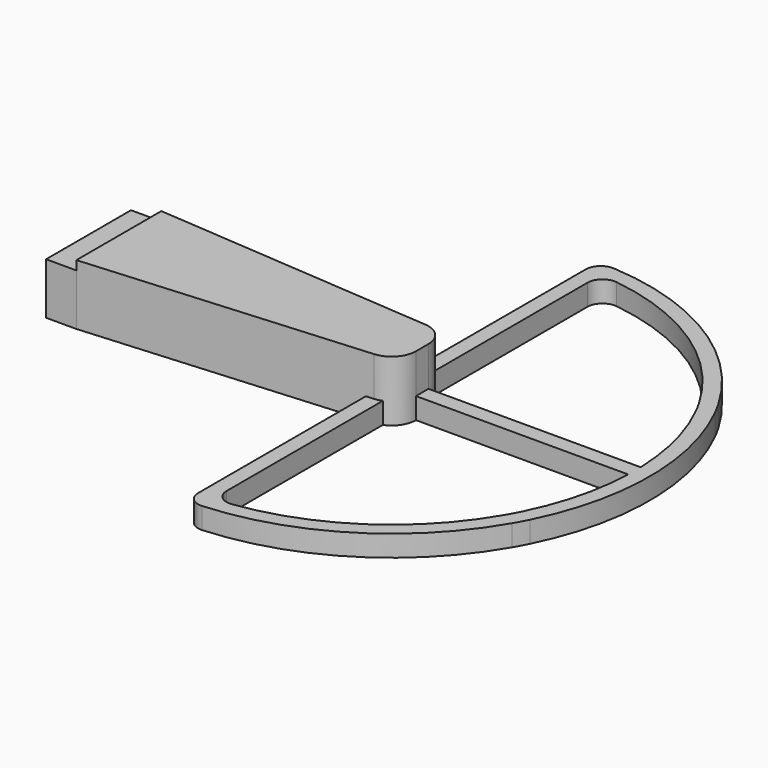
from build123d import *

# Parameters (mm, degrees)
F1_DEPTH = 10
F2_DEPTH = 17
F3_W     = 100
F3_H     = 35
F4_DEPTH = 3
F5_SIZE2 = 99.99999
F5_SIZE  = 7.49999
F6_R     = 8
F8_DEPTH = 7
F9_W     = 5.1550631039
F9_H     = 7


# Not quite as in the source:
# - a fillet or chamfer is up to 0.001 mm smaller than in the source, because OpenCascade refuses the exact size


with BuildPart() as f1:
    # F0 (on Top) → F1 (new body)
    with BuildSketch(Plane.XY):
        Polygon((-58.5, -8.5), (-58.5, -2.5), (-58.5, 0), (-58.5, 2.5), (-58.5, 8.5), (-63.5, 0), align=None)
        Polygon((-58.5, -2.5), (-55, -2.5), (-55, 2.5), (-58.5, 2.5), (-58.5, 0), align=None)
    extrude(amount=F1_DEPTH)

    # F0 (on Top) → F2 (join)
    with BuildSketch(Plane.XY):
        Polygon((-55, -17.5), (55, -17.5), (55, 17.5), (-55, 17.5), (-55, 2.5), (-55, -2.5), align=None)
    extrude(amount=F2_DEPTH)

    # F3 (on face) → F4 (join)
    with BuildSketch(Plane.XY.offset(17)):
        with Locations((5, 0)):
            Rectangle(F3_W, F3_H)
    extrude(amount=F4_DEPTH)

    # F5 (size 7.5 and 100 in the source; OpenCascade refuses exactly that, so slightly less here)
    f5_edges = [f1.edges().sort_by_distance(p)[0] for p in [
        (55, -17.5, 10),
        (55, 17.5, 10),
    ]]
    f5_side = f1.faces().sort_by_distance((55, 0, 10))[0]
    chamfer(f5_edges, length=F5_SIZE, length2=F5_SIZE2, reference=f5_side)

    # F6
    f6_edges = [f1.edges().sort_by_distance(p)[0] for p in [
        (55, -10.00001, 10),
        (55, 10.00001, 10),
    ]]
    fillet(f6_edges, radius=F6_R)

    # F7 (on face) → F8 (join)
    with BuildSketch(Plane.XY):
        with BuildLine():
            ThreePointArc((118.6121593217, 42.5), (89.7807277981, 72.2473973087), (50.3125, 84.8338219329))
            ThreePointArc((50.3125, 84.8338219329), (46.5767340156, 83.4879420476), (45, 79.8435971134))
            Line((45, 79.8435971134), (45, 0))
            Line((45, 0), (50, 2.8867513459))
            Line((50, 2.8867513459), (50, 74.3303437366))
            ThreePointArc((50, 74.3303437366), (51.708597057, 78.0942070001), (55.6666666667, 79.2856999857))
            ThreePointArc((55.6666666667, 79.2856999857), (89.5397594579, 66.4545696505), (114.2820323028, 40))
            Line((114.2820323028, 40), (118.6121593217, 42.5))
        make_face()
        with BuildLine():
            ThreePointArc((120.9846922835, 38.0962798523), (119.8308271392, 40.3155963576), (118.6121593217, 42.5))
            Line((118.6121593217, 42.5), (114.2820323028, 40))
            ThreePointArc((114.2820323028, 40), (115.4987732023, 37.8143223789), (116.6465834297, 35.5916715378))
            Line((116.6465834297, 35.5916715378), (120.9846922835, 38.0962798523))
        make_face()
        with BuildLine():
            ThreePointArc((120.9846922835, -38.0962798523), (130, 0), (120.9846922835, 38.0962798523))
            Line((120.9846922835, 38.0962798523), (116.6465834297, 35.5916715378))
            ThreePointArc((116.6465834297, 35.5916715378), (125, 0), (116.6465834297, -35.5916715378))
            Line((116.6465834297, -35.5916715378), (120.9846922835, -38.0962798523))
        make_face()
        with BuildLine():
            Line((50, -2.8867513459), (45, 0))
            Line((45, 0), (45, -79.8435971134))
            ThreePointArc((45, -79.8435971134), (46.5767340156, -83.4879420476), (50.3125, -84.8338219329))
            ThreePointArc((50.3125, -84.8338219329), (89.7807277981, -72.2473973087), (118.6121593217, -42.5))
            Line((118.6121593217, -42.5), (114.2820323028, -40))
            ThreePointArc((114.2820323028, -40), (89.5397594579, -66.4545696505), (55.6666666667, -79.2856999857))
            ThreePointArc((55.6666666667, -79.2856999857), (51.708597057, -78.0942070001), (50, -74.3303437366))
            Line((50, -74.3303437366), (50, -2.8867513459))
        make_face()
        Polygon((50, 2.8867513459), (45, 0), (50, -2.8867513459), align=None)
        with BuildLine():
            ThreePointArc((118.6121593217, -42.5), (119.8308271392, -40.3155963576), (120.9846922835, -38.0962798523))
            Line((120.9846922835, -38.0962798523), (116.6465834297, -35.5916715378))
            ThreePointArc((116.6465834297, -35.5916715378), (115.4987732023, -37.8143223789), (114.2820323028, -40))
            Line((114.2820323028, -40), (118.6121593217, -42.5))
        make_face()
    extrude(amount=F8_DEPTH)

    # F9 (on face) → F10 (join, up to the next surface of F1)
    with BuildSketch(Plane.YZ.offset(55)):
        with Locations((0, 3.5)):
            Rectangle(F9_W, F9_H)
    extrude(until=Until.NEXT)


solid = f1.part
